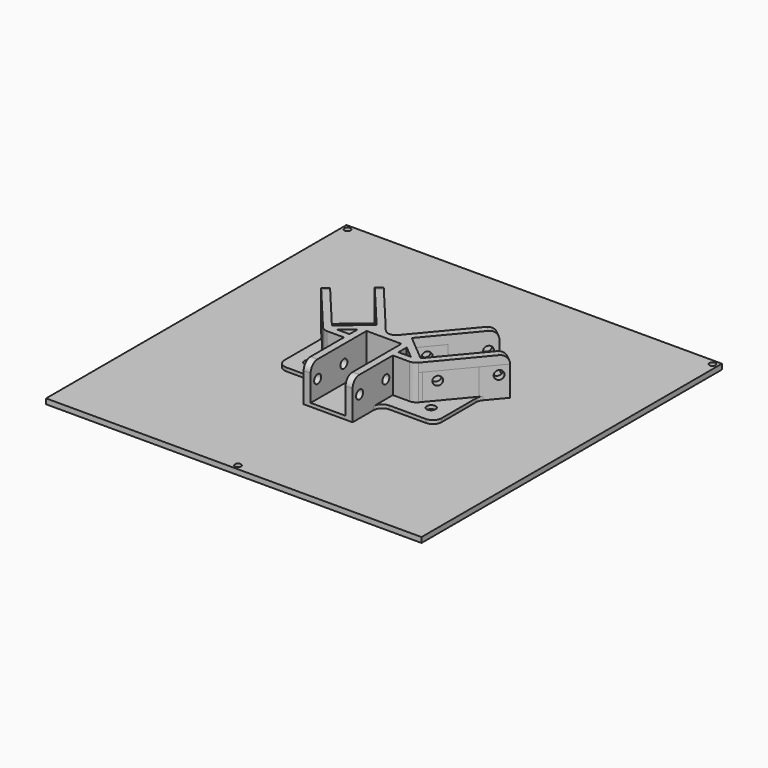
from build123d import *

# Parameters (mm, degrees)
F0_W          = 215
F0_H          = 215
F0_R          = 1.75
F1_DEPTH      = 3
F2_W          = 4
F2_H          = 20
F3_DEPTH      = 20
F2_R          = 5.5
F2_R_2        = 2.55
F2_W_2        = 20
F4_DEPTH      = 5
F5_R          = 2.5
F6_DEPTH      = 40
F7_R          = 2.5
F8_DEPTH      = 40
F9_R          = 2.5
F10_DEPTH     = 40
F11_T1_DEPTH  = 20
F11_T3_DEPTH  = 5
F11_T5_DEPTH  = 30
F11_T7_DEPTH  = 25.8367983923
F11_T9_DEPTH  = 29
F11_T11_DEPTH = 29
F11_T13_DEPTH = 29
F11_T15_DEPTH = 29
F11_T17_DEPTH = 29
F11_T19_DEPTH = 29


# Not quite as in the source:
# - a fillet or chamfer that OpenCascade refuses, or shapes differently, is made with other operations: its cross-section is extruded or revolved along the edge and cut away or added


with BuildPart() as f1:
    # F0 (on Top) → F1 (new body)
    with BuildSketch(Plane.XY):
        Rectangle(F0_W, F0_H)
        with Locations((0, -104.5)):
            Circle(F0_R, mode=Mode.SUBTRACT)
        with Locations((-104.5, 104.5)):
            Circle(F0_R, mode=Mode.SUBTRACT)
        with Locations((104.5, 104.5)):
            Circle(F0_R, mode=Mode.SUBTRACT)
    extrude(amount=F1_DEPTH)


with BuildPart() as f3:
    # F2 (on Top) → F3 (new body)
    with BuildSketch(Plane.XY):
        Polygon((-35.7447599302, 37.963242952), (-20.7037670278, 20), (-15.4867092456, 20), (-32.6778972141, 40.5311902024), align=None)
        with BuildLine():
            Line((-15.4867092456, 20), (-20.7037670278, 20))
            Line((-20.7037670278, 20), (-10.0652874269, 7.2946157909))
            Line((-10.0652874269, 7.2946157909), (-14, 4))
            Line((-14, 4), (-2.089580059, 4))
            Line((-2.089580059, 4), (-3.7261519654, 5.9545344482))
            ThreePointArc((-3.7261519654, 5.9545344482), (-4.2169362347, 6.4690725308), (-4.6372358245, 7.0426288856))
            Line((-4.6372358245, 7.0426288856), (-15.4867092456, 20))
        make_face()
        Polygon((-25.3996010074, -5.5451204608), (-45, 17.8633560503), (-45, 11.6326984705), (-28.4664637236, -8.1130677111), (-25.8985164732, -11.1799304272), (-21.1213736161, -7.1799304272), (-14, -1.2170577822), (-14, 0), (-14, 4), align=None)
        Polygon((-45, 11.6326984705), (-45, 17.8633560503), (-51.0790735108, 25.1235067004), (-54.1459362269, 22.55555945), align=None)
        Polygon((-2.089580059, 4), (-14, 4), (-14, 0), (-10, 0), (10, 0), (14, 0), (14, 4), (2.089580059, 4), align=None)
        Polygon((-21.1213736161, -7.1799304272), (-25.8985164732, -11.1799304272), (-14, -11.1799304272), (-14, -7.1799304272), align=None)
        Polygon((-10, 0), (-14, 0), (-14, -1.2170577822), (-14, -7.1799304272), (-14, -11.1799304272), (-14, -20), (-10, -20), align=None)
        Polygon((14, 0), (10, 0), (10, -20), (14, -20), (14, -11.1799304272), (14, -7.1799304272), (14, -1.2170577822), align=None)
        with Locations((12, -30)):
            Rectangle(F2_W, F2_H)
        with Locations((-12, -30)):
            Rectangle(F2_W, F2_H)
        Polygon((14, -7.1799304272), (14, -11.1799304272), (25.8985164732, -11.1799304272), (21.1213736161, -7.1799304272), align=None)
        Polygon((45, 11.6326984705), (45, 17.8633560503), (25.3996010074, -5.5451204608), (14, 4), (14, 0), (14, -1.2170577822), (21.1213736161, -7.1799304272), (25.8985164732, -11.1799304272), (28.4664637236, -8.1130677111), align=None)
        with BuildLine():
            Line((20.7037670278, 20), (15.4867092456, 20))
            Line((15.4867092456, 20), (4.6372358245, 7.0426288856))
            ThreePointArc((4.6372358245, 7.0426288856), (4.2169362347, 6.4690725308), (3.7261519654, 5.9545344482))
            Line((3.7261519654, 5.9545344482), (2.089580059, 4))
            Line((2.089580059, 4), (14, 4))
            Line((14, 4), (10.0652874269, 7.2946157909))
            Line((10.0652874269, 7.2946157909), (20.7037670278, 20))
        make_face()
        Polygon((32.6778972141, 40.5311902024), (15.4867092456, 20), (20.7037670278, 20), (35.7447599302, 37.963242952), align=None)
        Polygon((51.0790735108, 25.1235067004), (45, 17.8633560503), (45, 11.6326984705), (54.1459362269, 22.55555945), align=None)
    extrude(amount=F3_DEPTH)

    # F2 (on Top) + F3_face (on face) → F4 (join)
    with BuildSketch(Plane.XY):
        Polygon((-45, 17.8633560503), (-45, 20), (-20.7037670278, 20), (-35.7447599302, 37.963242952), (-51.0790735108, 25.1235067004), align=None)
        Polygon((-28.4664637236, -8.1130677111), (-45, 11.6326984705), (-45, -20), (-14, -20), (-14, -11.1799304272), (-25.8985164732, -11.1799304272), align=None)
        with Locations((-35, -10)):
            Circle(F2_R, mode=Mode.SUBTRACT)
        with Locations((-35, -10)):
            Circle(F2_R)
        with Locations((-35, -10)):
            Circle(F2_R_2, mode=Mode.SUBTRACT)
        Polygon((-14, -7.1799304272), (-14, -1.2170577822), (-21.1213736161, -7.1799304272), align=None)
        Polygon((-20.7037670278, 20), (-45, 20), (-45, 17.8633560503), (-25.3996010074, -5.5451204608), (-14, 4), (-10.0652874269, 7.2946157909), align=None)
        with Locations((0, -30)):
            Rectangle(F2_W_2, F2_H)
        Polygon((45, -20), (45, 11.6326984705), (28.4664637236, -8.1130677111), (25.8985164732, -11.1799304272), (14, -11.1799304272), (14, -20), align=None)
        with Locations((35, -10)):
            Circle(F2_R, mode=Mode.SUBTRACT)
        Polygon((21.1213736161, -7.1799304272), (14, -1.2170577822), (14, -7.1799304272), align=None)
        with Locations((35, -10)):
            Circle(F2_R)
        with Locations((35, -10)):
            Circle(F2_R_2, mode=Mode.SUBTRACT)
        Polygon((45, 20), (20.7037670278, 20), (10.0652874269, 7.2946157909), (14, 4), (25.3996010074, -5.5451204608), (45, 17.8633560503), align=None)
        with BuildLine():
            Line((15.4867092456, 20), (-15.4867092456, 20))
            Line((-15.4867092456, 20), (-4.6372358245, 7.0426288856))
            ThreePointArc((-4.6372358245, 7.0426288856), (-1.5403251224, 15.2799051618), (5.5, 10))
            ThreePointArc((5.5, 10), (5.2799051618, 8.4596748776), (4.6372358245, 7.0426288856))
            Line((4.6372358245, 7.0426288856), (15.4867092456, 20))
        make_face()
        with BuildLine():
            ThreePointArc((5.5, 10), (-1.5403251224, 15.2799051618), (-4.6372358245, 7.0426288856))
            Line((-4.6372358245, 7.0426288856), (-3.7261519654, 5.9545344482))
            ThreePointArc((-3.7261519654, 5.9545344482), (0, 4.5), (3.7261519654, 5.9545344482))
            Line((3.7261519654, 5.9545344482), (4.6372358245, 7.0426288856))
            ThreePointArc((4.6372358245, 7.0426288856), (5.2799051618, 8.4596748776), (5.5, 10))
        make_face()
        with Locations((0, 10)):
            Circle(F2_R_2, mode=Mode.SUBTRACT)
        with BuildLine():
            ThreePointArc((3.7261519654, 5.9545344482), (0, 4.5), (-3.7261519654, 5.9545344482))
            Line((-3.7261519654, 5.9545344482), (-2.089580059, 4))
            Line((-2.089580059, 4), (2.089580059, 4))
            Line((2.089580059, 4), (3.7261519654, 5.9545344482))
        make_face()
        Polygon((35.7447599302, 37.963242952), (20.7037670278, 20), (45, 20), (45, 17.8633560503), (51.0790735108, 25.1235067004), align=None)
        with Locations((0, -10)):
            Rectangle(F2_W_2, F2_H)
    with BuildSketch(Plane(origin=(0, 2.4667612993, 20), x_dir=(1, 0, 0), z_dir=(0, 0, 1))):
        with BuildLine():
            Line((-32.6778972141, 38.0644289031), (-35.7447599302, 35.4964816527))
            Line((-35.7447599302, 35.4964816527), (-10.0652874269, 4.8278544916))
            Line((-10.0652874269, 4.8278544916), (-25.3996010074, -8.0118817601))
            Line((-25.3996010074, -8.0118817601), (-51.0790735108, 22.6567454011))
            Line((-51.0790735108, 22.6567454011), (-54.1459362269, 20.0887981507))
            Line((-54.1459362269, 20.0887981507), (-25.8985164732, -13.6466917265))
            Line((-25.8985164732, -13.6466917265), (-14, -13.6466917265))
            Line((-14, -13.6466917265), (-14, -42.4667612993))
            Line((-14, -42.4667612993), (-10, -42.4667612993))
            Line((-10, -42.4667612993), (-10, -2.4667612993))
            Line((-10, -2.4667612993), (10, -2.4667612993))
            Line((10, -2.4667612993), (10, -42.4667612993))
            Line((10, -42.4667612993), (14, -42.4667612993))
            Line((14, -42.4667612993), (14, -13.6466917265))
            Line((14, -13.6466917265), (25.8985164732, -13.6466917265))
            Line((25.8985164732, -13.6466917265), (54.1459362269, 20.0887981507))
            Line((54.1459362269, 20.0887981507), (51.0790735108, 22.6567454011))
            Line((51.0790735108, 22.6567454011), (25.3996010074, -8.0118817601))
            Line((25.3996010074, -8.0118817601), (10.0652874269, 4.8278544916))
            Line((10.0652874269, 4.8278544916), (35.7447599302, 35.4964816527))
            Line((35.7447599302, 35.4964816527), (32.6778972141, 38.0644289031))
            Line((32.6778972141, 38.0644289031), (4.6372358245, 4.5758675863))
            ThreePointArc((4.6372358245, 4.5758675863), (4.2169362347, 4.0023112315), (3.7261519654, 3.4877731489))
            Line((3.7261519654, 3.4877731489), (2.089580059, 1.5332387007))
            Line((2.089580059, 1.5332387007), (-2.089580059, 1.5332387007))
            Line((-2.089580059, 1.5332387007), (-3.7261519654, 3.4877731489))
            ThreePointArc((-3.7261519654, 3.4877731489), (-4.2169362347, 4.0023112315), (-4.6372358245, 4.5758675863))
            Line((-4.6372358245, 4.5758675863), (-32.6778972141, 38.0644289031))
        make_face()
        Polygon((21.1213736161, -9.6466917265), (14, -9.6466917265), (14, -3.6838190815), align=None, mode=Mode.SUBTRACT)
        Polygon((-14, -9.6466917265), (-21.1213736161, -9.6466917265), (-14, -3.6838190815), align=None, mode=Mode.SUBTRACT)
    extrude(amount=F4_DEPTH)

    # F5 (on face) → F6 (cut)
    with BuildSketch(Plane.YZ.offset(14)):
        with Locations((-34.9799304272, 15)):
            Circle(F5_R)
        with Locations((-16.1799304272, 15)):
            Circle(F5_R)
    extrude(amount=-F6_DEPTH, mode=Mode.SUBTRACT)

    # F7 (on face) → F8 (cut)
    with BuildSketch(Plane(origin=(20.7275193584, -17.3555784101, 0), x_dir=(0.6419868126, 0.766715679, 0), z_dir=(0.766715679, -0.6419868126, 0))):
        with Locations((19.0546780923, 15)):
            Circle(F7_R)
        with Locations((47.0546780923, 15)):
            Circle(F7_R)
    extrude(amount=-F8_DEPTH, mode=Mode.SUBTRACT)

    # F9 (on face) → F10 (cut)
    with BuildSketch(Plane(origin=(-20.7275193584, -17.3555784101, 0), x_dir=(0.6419868126, -0.766715679, 0), z_dir=(-0.766715679, -0.6419868126, 0))):
        with Locations((-47.0546780923, 15)):
            Circle(F9_R)
        with Locations((-19.0546780923, 15)):
            Circle(F9_R)
    extrude(amount=-F10_DEPTH, mode=Mode.SUBTRACT)

    # F11: fillet of radius 5 on 18 edges, made by hand

    # F11_s2 → F11_t1 (join)
    with BuildSketch(Plane.XY.offset(5)):
        with BuildLine():
            ThreePointArc((3.5884390972, 5.7900659371), (1.870319244, 4.4695656767), (-0.2451392979, 4))
            Line((-0.2451392979, 4), (2.089580059, 4))
            Line((2.089580059, 4), (3.5884390972, 5.7900659371))
        make_face()
        with BuildLine():
            ThreePointArc((0.2451392979, 4), (-1.870319244, 4.4695656767), (-3.5884390972, 5.7900659371))
            Line((-3.5884390972, 5.7900659371), (-2.089580059, 4))
            Line((-2.089580059, 4), (0.2451392979, 4))
        make_face()
    extrude(amount=F11_T1_DEPTH)

    # F11_s4 → F11_t3 (join)
    with BuildSketch(Plane.XY):
        with BuildLine():
            ThreePointArc((-16.9855682838, 21.7900659371), (-15.2674484306, 20.4695656767), (-13.1519898887, 20))
            Line((-13.1519898887, 20), (-15.4867092456, 20))
            Line((-15.4867092456, 20), (-16.9855682838, 21.7900659371))
        make_face()
        with BuildLine():
            ThreePointArc((13.1519898887, 20), (15.2674484306, 20.4695656767), (16.9855682838, 21.7900659371))
            Line((16.9855682838, 21.7900659371), (15.4867092456, 20))
            Line((15.4867092456, 20), (13.1519898887, 20))
        make_face()
        with BuildLine():
            ThreePointArc((46.1664216049, 13.02573913), (45.300644088, 11.5234508184), (45, 9.8158050671))
            Line((45, 9.8158050671), (45, 11.6326984705))
            Line((45, 11.6326984705), (46.1664216049, 13.02573913))
        make_face()
        with BuildLine():
            ThreePointArc((14, -25), (15.4644660941, -21.4644660941), (19, -20))
            Line((19, -20), (14, -20))
            Line((14, -20), (14, -25))
        make_face()
        with BuildLine():
            ThreePointArc((-14, -25), (-15.4644660941, -21.4644660941), (-19, -20))
            Line((-19, -20), (-14, -20))
            Line((-14, -20), (-14, -25))
        make_face()
        with BuildLine():
            ThreePointArc((-46.1664216049, 13.02573913), (-45.300644088, 11.5234508184), (-45, 9.8158050671))
            Line((-45, 9.8158050671), (-45, 11.6326984705))
            Line((-45, 11.6326984705), (-46.1664216049, 13.02573913))
        make_face()
    extrude(amount=F11_T3_DEPTH)

    # F11_s6 → F11_t5 (cut)
    with BuildSketch(Plane.XY.offset(-12.5)):
        with BuildLine():
            ThreePointArc((-40, -20), (-43.5355339059, -18.5355339059), (-45, -15))
            Line((-45, -15), (-45, -20))
            Line((-45, -20), (-40, -20))
        make_face()
        with BuildLine():
            ThreePointArc((45, -15), (43.5355339059, -18.5355339059), (40, -20))
            Line((40, -20), (45, -20))
            Line((45, -20), (45, -15))
        make_face()
    extrude(amount=F11_T5_DEPTH, mode=Mode.SUBTRACT)

    # F11_s8 → F11_t7 (cut)
    with BuildSketch(Plane.XY.offset(5)):
        with BuildLine():
            ThreePointArc((-23.5637971163, -11.1799304272), (-25.6792556583, -10.7103647505), (-27.3973755114, -9.3898644901))
            Line((-27.3973755114, -9.3898644901), (-25.8985164732, -11.1799304272))
            Line((-25.8985164732, -11.1799304272), (-23.5637971163, -11.1799304272))
        make_face()
        with BuildLine():
            ThreePointArc((23.5637971163, -11.1799304272), (25.6792556583, -10.7103647505), (27.3973755114, -9.3898644901))
            Line((27.3973755114, -9.3898644901), (25.8985164732, -11.1799304272))
            Line((25.8985164732, -11.1799304272), (23.5637971163, -11.1799304272))
        make_face()
    extrude(amount=F11_T7_DEPTH, mode=Mode.SUBTRACT)

    # F11_s10 → F11_t9 (cut)
    with BuildSketch(Plane(origin=(10.3244656423, 8.6448874995, 0), x_dir=(0, 0, 1), z_dir=(-0.766715679, -0.6419868126, 0))):
        with BuildLine():
            ThreePointArc((20, 52.0546780923), (23.5355339059, 50.5902119982), (25, 47.0546780923))
            Line((25, 47.0546780923), (25, 52.0546780923))
            Line((25, 52.0546780923), (20, 52.0546780923))
        make_face()
    extrude(amount=F11_T9_DEPTH, mode=Mode.SUBTRACT)

    # F11_s12 → F11_t11 (cut)
    with BuildSketch(Plane(origin=(-8.0767106544, -6.7627960025, 0), x_dir=(0, 0, 1), z_dir=(-0.766715679, -0.6419868126, 0))):
        with BuildLine():
            ThreePointArc((20, 52.0546780923), (23.5355339059, 50.5902119982), (25, 47.0546780923))
            Line((25, 47.0546780923), (25, 52.0546780923))
            Line((25, 52.0546780923), (20, 52.0546780923))
        make_face()
    extrude(amount=F11_T11_DEPTH, mode=Mode.SUBTRACT)

    # F11_s14 → F11_t13 (cut)
    with BuildSketch(Plane.YZ.offset(-26.5)):
        with BuildLine():
            ThreePointArc((-40, 20), (-38.5355339059, 23.5355339059), (-35, 25))
            Line((-35, 25), (-40, 25))
            Line((-40, 25), (-40, 20))
        make_face()
    extrude(amount=F11_T13_DEPTH, mode=Mode.SUBTRACT)

    # F11_s16 → F11_t15 (cut)
    with BuildSketch(Plane.YZ.offset(-2.5)):
        with BuildLine():
            ThreePointArc((-40, 20), (-38.5355339059, 23.5355339059), (-35, 25))
            Line((-35, 25), (-40, 25))
            Line((-40, 25), (-40, 20))
        make_face()
    extrude(amount=F11_T15_DEPTH, mode=Mode.SUBTRACT)

    # F11_s18 → F11_t17 (cut)
    with BuildSketch(Plane(origin=(30.3114653462, -25.3804135674, 0), x_dir=(0, 0, 1), z_dir=(-0.766715679, 0.6419868126, 0))):
        with BuildLine():
            ThreePointArc((20, 52.0546780923), (23.5355339059, 50.5902119982), (25, 47.0546780923))
            Line((25, 47.0546780923), (25, 52.0546780923))
            Line((25, 52.0546780923), (20, 52.0546780923))
        make_face()
    extrude(amount=F11_T17_DEPTH, mode=Mode.SUBTRACT)

    # F11_s20 → F11_t19 (cut)
    with BuildSketch(Plane(origin=(11.9102890495, -9.9727300654, 0), x_dir=(0, 0, 1), z_dir=(-0.766715679, 0.6419868126, 0))):
        with BuildLine():
            ThreePointArc((20, 52.0546780923), (23.5355339059, 50.5902119982), (25, 47.0546780923))
            Line((25, 47.0546780923), (25, 52.0546780923))
            Line((25, 52.0546780923), (20, 52.0546780923))
        make_face()
    extrude(amount=F11_T19_DEPTH, mode=Mode.SUBTRACT)


solid = Compound([f1.part, f3.part])
